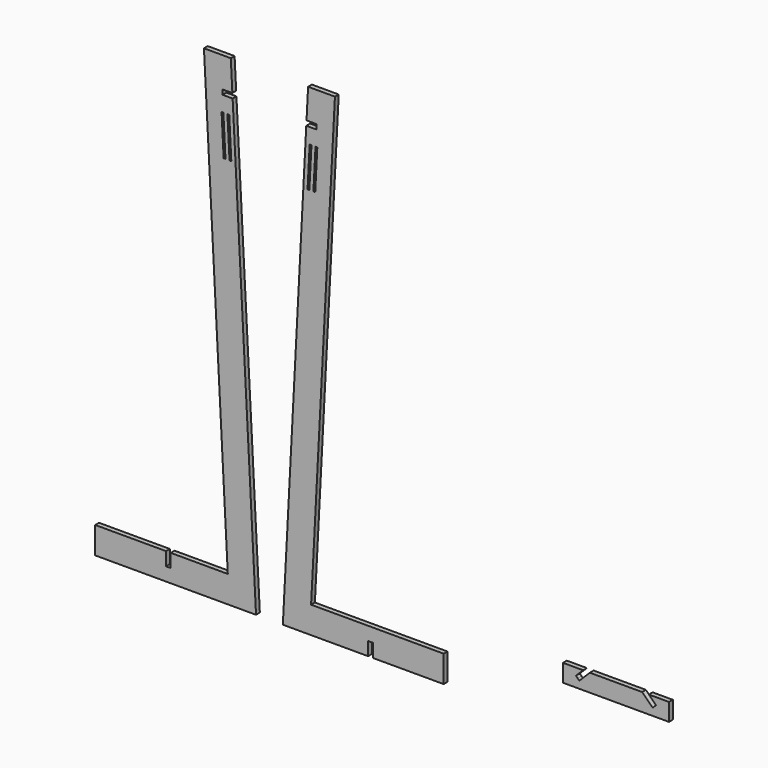
from build123d import *

# Parameters (mm, degrees)
F1_DEPTH = 18.034


# Not quite as in the source:
# - a feature names something its author has since deleted; it is built from what else it names


with BuildPart() as f1:
    # F0 (on Front) → F1 (new body)
    with BuildSketch(Plane.XZ):
        Polygon((502.5359392715, 0), (0, 0), (90.3873664019, 1724.6936931592), (39.5176512252, 1724.6936931592), (39.5176512252, 1267.4936931592), (-19.4161146469, 1267.4936931592), (-35.3129006397, 1267.4936931592), (-107.0640607285, -101.6), (216.2251596299, -101.6), (216.2251596299, -50.8), (234.2591596299, -50.8), (234.2591596299, -101.6), (502.5359392715, -101.6), align=None)
        Polygon((39.5176512252, 1267.4936931592), (39.5176512252, 1724.6936931592), (-11.3520639514, 1724.6936931592), (-17.3422731235, 1610.3936931592), (19.8126049849, 1610.3936931592), (19.8126049849, 1592.3596931592), (-18.2873950151, 1592.3596931592), (-24.6636398893, 1470.6936931592), (-8.7668538966, 1470.6936931592), (-5.4444328278, 1534.0892637075), (1.422978721, 1534.0892637075), (-1.8994423478, 1470.6936931592), (13.4581461034, 1470.6936931592), (16.7805671722, 1534.0892637075), (23.647978721, 1534.0892637075), (20.3255576522, 1470.6936931592), (28.9262730809, 1470.6936931592), (28.9262730809, 1445.2936931592), (18.9944000584, 1445.2936931592), (15.6531687901, 1381.539202623), (8.8045674408, 1381.8981226109), (12.1269885096, 1445.2936931592), (-3.2305999416, 1445.2936931592), (-6.5718312099, 1381.539202623), (-13.4204325592, 1381.8981226109), (-19.4161146469, 1267.4936931592), align=None)
        Polygon((-35.3129006397, 1267.4936931592), (-19.4161146469, 1267.4936931592), (-13.4204325592, 1381.8981226109), (-10.0980114904, 1445.2936931592), (-25.9947974831, 1445.2936931592), align=None)
        Polygon((-8.7668538966, 1470.6936931592), (-24.6636398893, 1470.6936931592), (-25.7346158366, 1450.2582547212), (-10.0980114904, 1445.2936931592), (-9.4230275025, 1458.1731548939), align=None)
        Polygon((-25.7346158366, 1450.2582547212), (-25.9947974831, 1445.2936931592), (-10.0980114904, 1445.2936931592), align=None)
        Polygon((-2.5744262358, 1457.8142333288), (-3.2305999416, 1445.2936931592), (12.1269885096, 1445.2936931592), (12.8019724807, 1458.173154574), (13.4581461034, 1470.6936931592), (-1.8994423478, 1470.6936931592), align=None)
        Polygon((19.6505737569, 1457.8142331896), (18.9944000584, 1445.2936931592), (28.9262730809, 1445.2936931592), (28.9262730809, 1470.6936931592), (20.3255576522, 1470.6936931592), align=None)
    extrude(amount=F1_DEPTH)


with BuildPart() as f1b:
    # F0 (on Front) → F1, piece 2 (new body)
    with BuildSketch(Plane.XZ):
        Polygon((954.8041553716, 50.0226186452), (964.3706549533, 50.0226186452), (977.1226186452, 62.7745823371), (1004.0633870084, 89.7153507003), (1031.0041553716, 116.6561190635), (954.8041553716, 116.6561190635), align=None)
        Polygon((977.1226186452, 62.7745823371), (964.3706549533, 50.0226186452), (989.8745823371, 50.0226186452), (983.4986004912, 56.3986004912), align=None)
        Polygon((983.4986004912, 56.3986004912), (989.8745823371, 50.0226186452), (1016.8153507003, 76.9633870084), (1010.4393688544, 83.3393688544), (1004.0633870084, 89.7153507003), (977.1226186452, 62.7745823371), align=None)
        Polygon((1016.8153507003, 76.9633870084), (989.8745823371, 50.0226186452), (1155.7, 50.0226186452), (1321.5254176629, 50.0226186452), (1294.5846492997, 76.9633870084), (1254.8919172446, 116.6561190635), (1155.7, 116.6561190635), (1056.5080827554, 116.6561190635), align=None)
        Polygon((1294.5846492997, 76.9633870084), (1321.5254176629, 50.0226186452), (1347.0293450467, 50.0226186452), (1307.3366129916, 89.7153507003), (1300.9606311456, 83.3393688544), align=None)
        Polygon((1307.3366129916, 89.7153507003), (1347.0293450467, 50.0226186452), (1356.5958446284, 50.0226186452), (1356.5958446284, 116.6561190635), (1280.3958446284, 116.6561190635), align=None)
    extrude(amount=F1_DEPTH)


with BuildPart() as f1c:
    # F0 (on Front) → F1, piece 3 (new body)
    with BuildSketch(Plane.XZ):
        Polygon((-531.953281087, 0), (-531.953281087, -50.8), (-549.987281087, -50.8), (-549.987281087, 0), (-818.2640607285, 0), (-818.2640607285, -101.6), (-208.6640607285, -101.6), (-297.440726442, 1592.3596931592), (-335.540726442, 1592.3596931592), (-335.540726442, 1610.3936931592), (-298.3858483336, 1610.3936931592), (-304.3760575056, 1724.6936931592), (-406.115487859, 1724.6936931592), (-315.7281214571, 0), align=None)
        Polygon((-324.5326888979, 1381.8981226109), (-331.3812902472, 1381.539202623), (-339.3761001781, 1534.0892637075), (-332.5086886293, 1534.0892637075), align=None, mode=Mode.SUBTRACT)
        Polygon((-317.1511001781, 1534.0892637075), (-310.2836886293, 1534.0892637075), (-302.3076888979, 1381.8981226109), (-309.1562902472, 1381.539202623), align=None, mode=Mode.SUBTRACT)
    extrude(amount=F1_DEPTH)


solid = Compound([f1.part, f1b.part, f1c.part])
